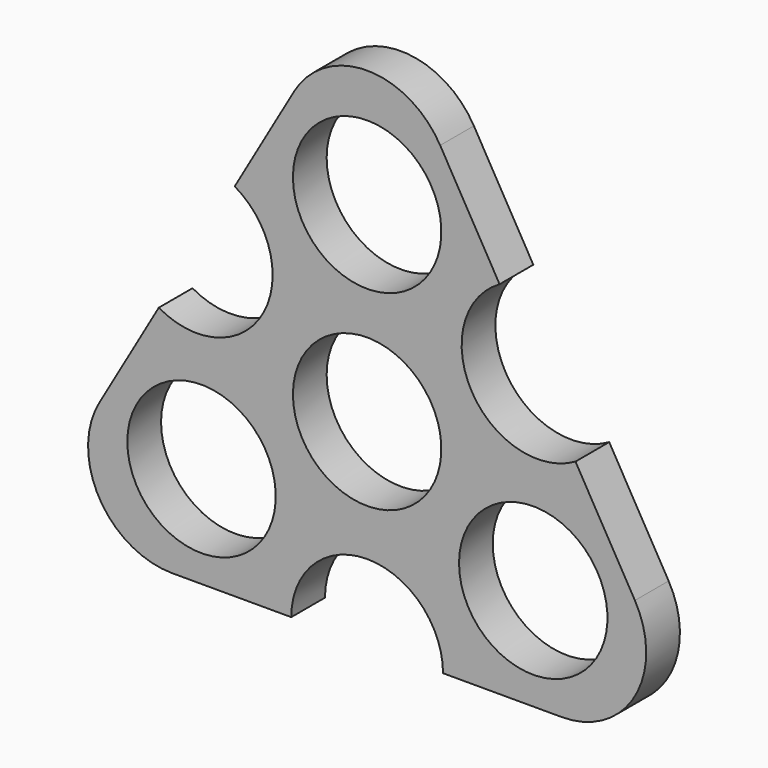
from build123d import *

# Parameters (mm, degrees)
F1_DEPTH = 6.35
F4_R     = 11.176
F5_DEPTH = 25.4
F6_R     = 12.7
F7_R     = 11.176
F8_DEPTH = 25.4


# Not quite as in the source:
# - a feature of the source that left no trace in its solid (it failed there, or was rolled back) is left out


with BuildPart() as f1:
    # F0 (on Front) → F1 (new body)
    with BuildSketch(Plane.XZ):
        with BuildLine():
            Line((19.9482194655, 24.7153370319), (0, 59.2666666667))
            Line((0, 59.2666666667), (-19.9482194655, 24.7153370319))
            ThreePointArc((-19.9482194655, 24.7153370319), (-15.7645491002, 20.5316666667), (-14.2332194655, 14.8166666667))
            ThreePointArc((-14.2332194655, 14.8166666667), (-19.9482194655, 4.9179963014), (-31.3782194655, 4.9179963014))
            Line((-31.3782194655, 4.9179963014), (-51.326438931, -29.6333333333))
            Line((-51.326438931, -29.6333333333), (-11.43, -29.6333333333))
            ThreePointArc((-11.43, -29.6333333333), (0, -18.2033333333), (11.43, -29.6333333333))
            Line((11.43, -29.6333333333), (51.326438931, -29.6333333333))
            Line((51.326438931, -29.6333333333), (31.3782194655, 4.9179963014))
            ThreePointArc((31.3782194655, 4.9179963014), (15.7645491002, 9.1016666667), (19.9482194655, 24.7153370319))
        make_face()
    extrude(amount=F1_DEPTH)

    # F4 (on face) → F5 (cut)
    with BuildSketch(Plane(origin=(0, 0, 0), x_dir=(-1, 0, 0), z_dir=(0, 1, 0))):
        with Locations((0, 28.7866666667)):
            Circle(F4_R)
        with Locations((-25.0159751206, -14.245354451)):
            Circle(F4_R)
        with Locations((24.9412614338, -14.3738179923)):
            Circle(F4_R)
    extrude(amount=-F5_DEPTH, mode=Mode.SUBTRACT)

    # F6
    f6_edges = [f1.edges().sort_by_distance(p)[0] for p in [
        (0, -3.175, 59.266667),
        (51.326439, -3.175, -29.633333),
        (-51.326439, -3.175, -29.633333),
    ]]
    fillet(f6_edges, radius=F6_R)

    # F7 (on face) → F8 (cut)
    with BuildSketch(Plane(origin=(0, 0, 0), x_dir=(-1, 0, 0), z_dir=(0, 1, 0))):
        Circle(F7_R)
    extrude(amount=-F8_DEPTH, mode=Mode.SUBTRACT)


solid = f1.part
